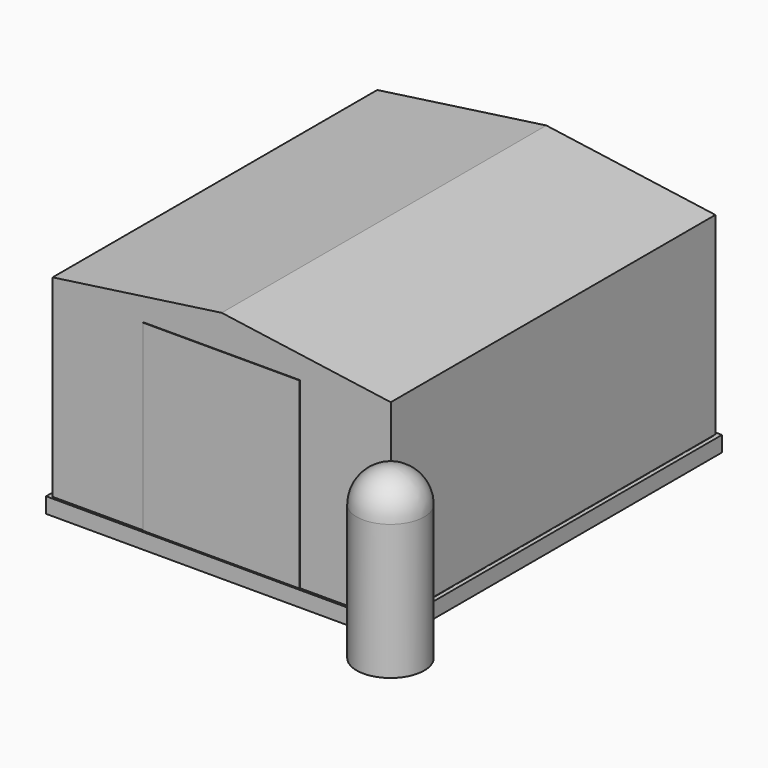
from build123d import *

# Parameters (mm, degrees)
F0_W     = 3130.55
F0_H     = 3702.05
F0_W_2   = 3054.35
F0_H_2   = 38.1
F1_DEPTH = 139.7
F2_W     = 3048
F2_H     = 3657.6
F3_DEPTH = 1955.8
F4_SIZE2 = 214.184222
F4_SIZE  = 1523.99999
F5_W     = 1409.7
F5_H     = 1651
F6_DEPTH = 6.35
F7_R     = 304.8
F8_DEPTH = 1524
F9_R     = 304.8


# Not quite as in the source:
# - a fillet or chamfer is up to 0.001 mm smaller than in the source, because OpenCascade refuses the exact size


with BuildPart() as f1:
    # F0 (on Top) → F1 (new body)
    with BuildSketch(Plane.XY):
        Rectangle(F0_W, F0_H)
        Polygon((1527.175, -1492.25), (1527.175, -1812.925), (-1527.175, -1812.925), (-1527.175, -1492.25), (-1527.175, -1454.15), (-1527.175, -1123.95), (-1527.175, -1085.85), (-1527.175, -755.65), (-1527.175, -717.55), (-1527.175, -387.35), (-1527.175, -349.25), (-1527.175, -19.05), (-1527.175, 19.05), (-1527.175, 349.25), (-1527.175, 387.35), (-1527.175, 717.55), (-1527.175, 755.65), (-1527.175, 1085.85), (-1527.175, 1123.95), (-1527.175, 1454.15), (-1527.175, 1492.25), (-1527.175, 1812.925), (1527.175, 1812.925), (1527.175, 1492.25), (1527.175, 1454.15), (1527.175, 1123.95), (1527.175, 1085.85), (1527.175, 755.65), (1527.175, 717.55), (1527.175, 387.35), (1527.175, 349.25), (1527.175, 19.05), (1527.175, -19.05), (1527.175, -349.25), (1527.175, -387.35), (1527.175, -717.55), (1527.175, -755.65), (1527.175, -1085.85), (1527.175, -1123.95), (1527.175, -1454.15), align=None, mode=Mode.SUBTRACT)
        with Locations((0, -368.3)):
            Rectangle(F0_W_2, F0_H_2)
        with Locations((0, -736.6)):
            Rectangle(F0_W_2, F0_H_2)
        with Locations((0, -1104.9)):
            Rectangle(F0_W_2, F0_H_2)
        with Locations((0, -1473.2)):
            Rectangle(F0_W_2, F0_H_2)
        Rectangle(F0_W_2, F0_H_2)
        with Locations((0, 368.3)):
            Rectangle(F0_W_2, F0_H_2)
        with Locations((0, 736.6)):
            Rectangle(F0_W_2, F0_H_2)
        with Locations((0, 1104.9)):
            Rectangle(F0_W_2, F0_H_2)
        with Locations((0, 1473.2)):
            Rectangle(F0_W_2, F0_H_2)
    extrude(amount=-F1_DEPTH)


with BuildPart() as f3:
    # F2 (on Top) → F3 (new body)
    with BuildSketch(Plane.XY):
        Rectangle(F2_W, F2_H)
    extrude(amount=F3_DEPTH)

    # F4 (size 1524 and 214.1842320864 in the source; OpenCascade refuses exactly that, so slightly less here)
    f4_edges = [f3.edges().sort_by_distance(p)[0] for p in [
        (1524, 0, 1955.8),
        (-1524, 0, 1955.8),
    ]]
    f4_side = f3.faces().sort_by_distance((0, 0, 1955.8))[0]
    chamfer(f4_edges, length=F4_SIZE, length2=F4_SIZE2, reference=f4_side)


with BuildPart() as f6:
    # F5 (on face) → F6 (new body)
    with BuildSketch(Plane.XZ.offset(1828.8)):
        with Locations((0, 825.5)):
            Rectangle(F5_W, F5_H)
    extrude(amount=F6_DEPTH)


with BuildPart() as f8:
    # F7 (on Top) → F8 (new body)
    with BuildSketch(Plane.XY):
        with Locations((1868.3955669403, -2262.4032497406)):
            Circle(F7_R)
    extrude(amount=F8_DEPTH)

    # F9
    f9_edges = [f8.edges().sort_by_distance(p)[0] for p in [
        (1563.595567, -2262.40325, 1524),
    ]]
    fillet(f9_edges, radius=F9_R)


solid = Compound([f1.part, f3.part, f6.part, f8.part])
